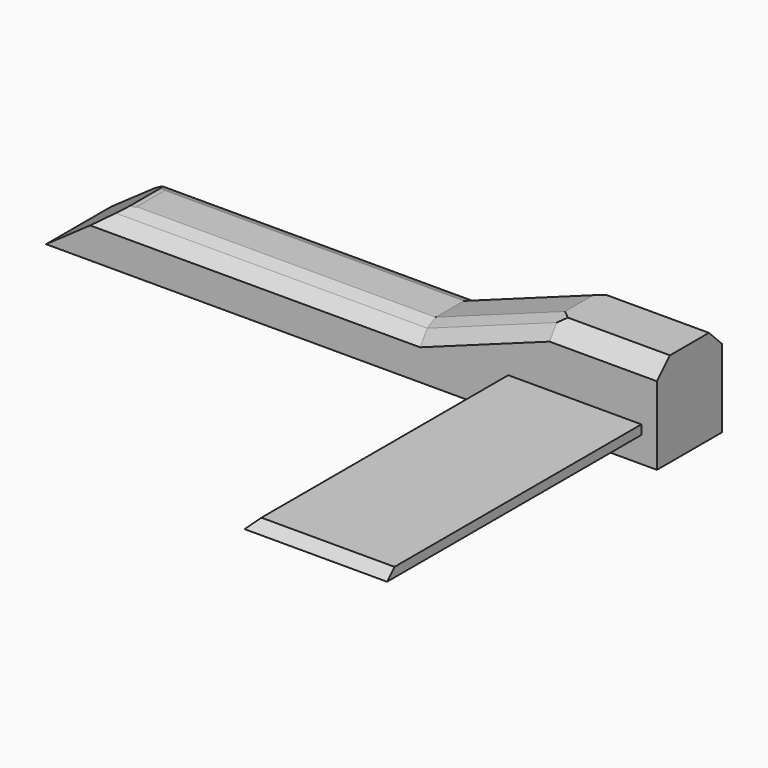
from build123d import *

# Parameters (mm, degrees)
F0_W         = 23.517049849
F0_H         = 14.5949013531
F1_DEPTH     = 25.4
F2_T4_DEPTH  = 242.6459393762
F3_SIZE      = 5.08
F4_T1_DEPTH  = 127.9476749925
F5_W         = 46.7211659998
F5_H         = 2.9200753197
F6_DEPTH     = 127
F7_T1_DEPTH  = 114.6641495789
F7_T3_DEPTH  = 72.8494651575
F7_T8_DEPTH  = 58.5750464118
F7_T14_DEPTH = 58.5750464118
F7_T20_DEPTH = 58.5750464118
F7_T26_DEPTH = 104.9770798243
F7_T32_DEPTH = 104.9770798243
F7_T38_DEPTH = 104.9770798243
F7_T44_DEPTH = 104.9770798243
F7_T50_DEPTH = 104.9770798243
F7_T56_DEPTH = 104.9770798243
F7_T62_DEPTH = 58.5750464118
F7_T68_DEPTH = 58.5750464118
F7_T74_DEPTH = 58.5750464118
F7_T81_DEPTH = 104.9770798243
F7_T86_DEPTH = 58.5750464118
F7_T94_DEPTH = 104.9770798243
F7_T99_DEPTH = 58.5750464118


# Not quite as in the source:
# - a fillet or chamfer that OpenCascade refuses, or shapes differently, is made with other operations: its cross-section is extruded or revolved along the edge and cut away or added


with BuildPart() as f1:
    # F0 (on Front) → F1 (new body)
    with BuildSketch(Plane.XZ):
        with Locations((-103.8943566382, 7.2974506766)):
            Rectangle(F0_W, F0_H)
        Polygon((-92.1358317137, 0), (0, 0), (0, 14.7395525128), (-92.1358317137, 14.7395525128), (-92.1358317137, 14.5949013531), align=None)
        Polygon((0, 0), (76.3533711433, 0), (76.3533711433, 29.4791050255), (0, 29.4791050255), (0, 14.7395525128), align=None)
    extrude(amount=F1_DEPTH)

    # F2: chamfer of 15.24 x 41.8715558725 on 1 edges, made by hand


with BuildPart() as f2_tool2:
    # F2_s3 → F2_t4 (new body)
    with BuildSketch(Plane.XZ.offset(-108.6229696881)):
        Polygon((41.8715558725, 29.4791050255), (0, 14.2391050255), (0, 29.4791050255), align=None)
    extrude(amount=F2_T4_DEPTH)

    split(bisect_by=Plane.XY.offset(14.7395525128), keep=Keep.TOP)


with BuildPart() as f1_1:
    add(f1.part)

    # F2_t1: cut F2_tool2
    add(f2_tool2.part, mode=Mode.SUBTRACT)

    # F3
    f3_edges = [f1_1.edges().sort_by_distance(p)[0] for p in [
        (-45.380432, -25.4, 14.739553),
        (-45.380432, 0, 14.739553),
        (59.112464, -25.4, 29.479105),
        (21.623262, -25.4, 22.109329),
        (21.623262, 0, 22.109329),
        (59.112464, 0, 29.479105),
    ]]
    chamfer(f3_edges, length=F3_SIZE)

    # F4: chamfer of 15.24 x 21.7649756227 on 1 edges, made by hand

    # F4_s2 → F4_t1 (cut)
    with BuildSketch(Plane.XZ.offset(-51.2738374963)):
        Polygon((-115.6528815627, -0.6450986469), (-93.88790594, 14.5949013531), (-115.6528815627, 14.5949013531), align=None)
    extrude(amount=F4_T1_DEPTH, mode=Mode.SUBTRACT)

    # F5 (on face) → F6 (join)
    with BuildSketch(Plane(origin=(0, 0, 0), x_dir=(-1, 0, 0), z_dir=(0, 1, 0))):
        with Locations((-48.1185736135, 9.490238037)):
            Rectangle(F5_W, F5_H)
    extrude(amount=-F6_DEPTH)

    # F7: chamfer of 5.08 on 6 edges, made by hand

    # F7_s2 → F7_t1 (cut)
    with BuildSketch(Plane.XZ.offset(25.4)):
        with BuildLine():
            Line((29.9816747115, 11.0939597948), (24.6143065156, 5.7265915989))
            Line((24.6143065156, 5.7265915989), (24.5127065156, 5.7265915989))
            ThreePointArc((24.5127065156, 5.7265915989), (24.6563906136, 8.3384336478), (24.6563906136, 10.9502756968))
            Line((24.6563906136, 10.9502756968), (24.7579906136, 11.0518756968))
            ThreePointArc((24.7579906136, 11.0518756968), (27.3698326625, 11.0518756968), (29.9816747115, 11.1955597948))
            Line((29.9816747115, 11.1955597948), (29.9816747115, 11.0939597948))
        make_face()
    extrude(amount=F7_T1_DEPTH, mode=Mode.SUBTRACT)

    # F7_s4 → F7_t3 (cut)
    with BuildSketch(Plane.YZ.offset(11.6938410347)):
        with BuildLine():
            Line((-121.7763159021, 11.0939597948), (-127.1436840979, 5.7265915989))
            Line((-127.1436840979, 5.7265915989), (-127.2452840979, 5.7265915989))
            ThreePointArc((-127.2452840979, 5.7265915989), (-127.1016, 8.3384336478), (-127.1016, 10.9502756968))
            Line((-127.1016, 10.9502756968), (-127, 11.0518756968))
            ThreePointArc((-127, 11.0518756968), (-124.388157951, 11.0518756968), (-121.7763159021, 11.1955597948))
            Line((-121.7763159021, 11.1955597948), (-121.7763159021, 11.0939597948))
        make_face()
    extrude(amount=F7_T3_DEPTH, mode=Mode.SUBTRACT)


with BuildPart() as f7_tool6:
    # F7_s7 → F7_t8 (new body)
    with BuildSketch(Plane(origin=(0.563938989, 0, 0.2052570059), x_dir=(0, 1, 0), z_dir=(0.9396926208, 0, 0.3420201433))):
        with BuildLine():
            Line((-7.3719372179, 13.4581431925), (-3.4043701274, 11.814723094))
            Line((-3.4043701274, 11.814723094), (-3.3325280785, 11.886565143))
            ThreePointArc((-3.3325280785, 11.886565143), (-4.1978357766, 12.6419017936), (-5.008157951, 13.452223968))
            Line((-5.008157951, 13.452223968), (-5.08, 13.4819819191))
            ThreePointArc((-5.08, 13.4819819191), (-6.2259686089, 13.4819819191), (-7.3719372179, 13.5597431925))
            Line((-7.3719372179, 13.5597431925), (-7.3719372179, 13.4581431925))
        make_face()
    extrude(amount=F7_T8_DEPTH)

    split(bisect_by=Plane.XY.offset(14.7395525128), keep=Keep.BOTTOM)

    split(bisect_by=Plane(origin=(0, 4.8297762564, 4.8297762564), x_dir=(1, 0, 0), z_dir=(0, 0.7071067812, 0.7071067812)), keep=Keep.TOP)


with BuildPart() as f1_2:
    add(f1_1.part)

    # F7_t5: cut F7_tool6
    add(f7_tool6.part, mode=Mode.SUBTRACT)


with BuildPart() as f7_tool12:
    # F7_s13 → F7_t14 (new body)
    with BuildSketch(Plane(origin=(0.563938989, 0, 0.2052570059), x_dir=(0, 1, 0), z_dir=(0.9396926208, 0, 0.3420201433))):
        with BuildLine():
            Line((-7.3719372179, 13.4581431925), (-3.4043701274, 11.814723094))
            Line((-3.4043701274, 11.814723094), (-3.3325280785, 11.886565143))
            ThreePointArc((-3.3325280785, 11.886565143), (-4.1978357766, 12.6419017936), (-5.008157951, 13.452223968))
            Line((-5.008157951, 13.452223968), (-5.08, 13.4819819191))
            ThreePointArc((-5.08, 13.4819819191), (-6.2259686089, 13.4819819191), (-7.3719372179, 13.5597431925))
            Line((-7.3719372179, 13.5597431925), (-7.3719372179, 13.4581431925))
        make_face()
    extrude(amount=F7_T14_DEPTH)

    split(bisect_by=Plane.XY.offset(14.7395525128), keep=Keep.TOP)

    split(bisect_by=Plane(origin=(0, 4.8297762564, 4.8297762564), x_dir=(1, 0, 0), z_dir=(0, -0.7071067812, -0.7071067812)), keep=Keep.TOP)


with BuildPart() as f1_3:
    add(f1_2.part)

    # F7_t11: cut F7_tool12
    add(f7_tool12.part, mode=Mode.SUBTRACT)


with BuildPart() as f7_tool18:
    # F7_s19 → F7_t20 (new body)
    with BuildSketch(Plane(origin=(0.563938989, 0, 0.2052570059), x_dir=(0, 1, 0), z_dir=(0.9396926208, 0, 0.3420201433))):
        with BuildLine():
            Line((-7.3719372179, 13.4581431925), (-3.4043701274, 11.814723094))
            Line((-3.4043701274, 11.814723094), (-3.3325280785, 11.886565143))
            ThreePointArc((-3.3325280785, 11.886565143), (-4.1978357766, 12.6419017936), (-5.008157951, 13.452223968))
            Line((-5.008157951, 13.452223968), (-5.08, 13.4819819191))
            ThreePointArc((-5.08, 13.4819819191), (-6.2259686089, 13.4819819191), (-7.3719372179, 13.5597431925))
            Line((-7.3719372179, 13.5597431925), (-7.3719372179, 13.4581431925))
        make_face()
    extrude(amount=F7_T20_DEPTH)

    split(bisect_by=Plane.XY.offset(14.7395525128), keep=Keep.TOP)

    split(bisect_by=Plane(origin=(0, 4.8297762564, 4.8297762564), x_dir=(1, 0, 0), z_dir=(0, 0.7071067812, 0.7071067812)), keep=Keep.TOP)


with BuildPart() as f1_4:
    add(f1_3.part)

    # F7_t17: cut F7_tool18
    add(f7_tool18.part, mode=Mode.SUBTRACT)


with BuildPart() as f7_tool24:
    # F7_s25 → F7_t26 (new body)
    with BuildSketch(Plane.YZ.offset(-97.8689716836)):
        with BuildLine():
            Line((-7.3719372179, 14.8173137862), (-3.4043701274, 13.1738936877))
            Line((-3.4043701274, 13.1738936877), (-3.3325280785, 13.2457357367))
            ThreePointArc((-3.3325280785, 13.2457357367), (-4.1978357766, 14.0010723873), (-5.008157951, 14.8113945617))
            Line((-5.008157951, 14.8113945617), (-5.08, 14.8411525128))
            ThreePointArc((-5.08, 14.8411525128), (-6.2259686089, 14.8411525128), (-7.3719372179, 14.9189137862))
            Line((-7.3719372179, 14.9189137862), (-7.3719372179, 14.8173137862))
        make_face()
    extrude(amount=F7_T26_DEPTH)

    split(bisect_by=Plane(origin=(-4.5763601417, 0, 12.5734461526), x_dir=(0, 1, 0), z_dir=(-0.3420201433, 0, 0.9396926208)), keep=Keep.TOP)

    split(bisect_by=Plane(origin=(-1.4194489068, 4.1501909595, 3.8999038195), x_dir=(-0.9461886483, -0.3236155771, 0), z_dir=(-0.2418447626, 0.7071067812, 0.6644630244)), keep=Keep.TOP)


with BuildPart() as f1_5:
    add(f1_4.part)

    # F7_t23: cut F7_tool24
    add(f7_tool24.part, mode=Mode.SUBTRACT)


with BuildPart() as f7_tool30:
    # F7_s31 → F7_t32 (new body)
    with BuildSketch(Plane.YZ.offset(-97.8689716836)):
        with BuildLine():
            Line((-7.3719372179, 14.8173137862), (-3.4043701274, 13.1738936877))
            Line((-3.4043701274, 13.1738936877), (-3.3325280785, 13.2457357367))
            ThreePointArc((-3.3325280785, 13.2457357367), (-4.1978357766, 14.0010723873), (-5.008157951, 14.8113945617))
            Line((-5.008157951, 14.8113945617), (-5.08, 14.8411525128))
            ThreePointArc((-5.08, 14.8411525128), (-6.2259686089, 14.8411525128), (-7.3719372179, 14.9189137862))
            Line((-7.3719372179, 14.9189137862), (-7.3719372179, 14.8173137862))
        make_face()
    extrude(amount=F7_T32_DEPTH)

    split(bisect_by=Plane(origin=(-4.5763601417, 0, 12.5734461526), x_dir=(0, 1, 0), z_dir=(0.3420201433, 0, -0.9396926208)), keep=Keep.TOP)

    split(bisect_by=Plane(origin=(-1.4194489068, 4.1501909595, 3.8999038195), x_dir=(-0.9461886483, -0.3236155771, 0), z_dir=(-0.2418447626, 0.7071067812, 0.6644630244)), keep=Keep.TOP)


with BuildPart() as f1_6:
    add(f1_5.part)

    # F7_t29: cut F7_tool30
    add(f7_tool30.part, mode=Mode.SUBTRACT)


with BuildPart() as f7_tool36:
    # F7_s37 → F7_t38 (new body)
    with BuildSketch(Plane.YZ.offset(-97.8689716836)):
        with BuildLine():
            Line((-7.3719372179, 14.8173137862), (-3.4043701274, 13.1738936877))
            Line((-3.4043701274, 13.1738936877), (-3.3325280785, 13.2457357367))
            ThreePointArc((-3.3325280785, 13.2457357367), (-4.1978357766, 14.0010723873), (-5.008157951, 14.8113945617))
            Line((-5.008157951, 14.8113945617), (-5.08, 14.8411525128))
            ThreePointArc((-5.08, 14.8411525128), (-6.2259686089, 14.8411525128), (-7.3719372179, 14.9189137862))
            Line((-7.3719372179, 14.9189137862), (-7.3719372179, 14.8173137862))
        make_face()
    extrude(amount=F7_T38_DEPTH)

    split(bisect_by=Plane(origin=(-4.5763601417, 0, 12.5734461526), x_dir=(0, 1, 0), z_dir=(-0.3420201433, 0, 0.9396926208)), keep=Keep.TOP)

    split(bisect_by=Plane(origin=(-1.4194489068, 4.1501909595, 3.8999038195), x_dir=(0.9461886483, 0.3236155771, 0), z_dir=(0.2418447626, -0.7071067812, -0.6644630244)), keep=Keep.TOP)


with BuildPart() as f1_7:
    add(f1_6.part)

    # F7_t35: cut F7_tool36
    add(f7_tool36.part, mode=Mode.SUBTRACT)


with BuildPart() as f7_tool42:
    # F7_s43 → F7_t44 (new body)
    with BuildSketch(Plane.YZ.offset(7.1081081408)):
        with BuildLine():
            Line((-21.9956298726, 13.1738936877), (-18.0280627821, 14.8173137862))
            Line((-18.0280627821, 14.8173137862), (-18.0280627821, 14.9189137862))
            ThreePointArc((-18.0280627821, 14.9189137862), (-19.1740313911, 14.8411525128), (-20.32, 14.8411525128))
            Line((-20.32, 14.8411525128), (-20.391842049, 14.8113945617))
            ThreePointArc((-20.391842049, 14.8113945617), (-21.2021642234, 14.0010723873), (-22.0674719215, 13.2457357367))
            Line((-22.0674719215, 13.2457357367), (-21.9956298726, 13.1738936877))
        make_face()
    extrude(amount=-F7_T44_DEPTH)

    split(bisect_by=Plane(origin=(-5.763104727, -16.8501909595, 15.8340001035), x_dir=(-0.9461886483, 0.3236155771, 0), z_dir=(0.2418447626, 0.7071067812, -0.6644630244)), keep=Keep.TOP)

    split(bisect_by=Plane(origin=(-4.5763601417, 0, 12.5734461526), x_dir=(0, 1, 0), z_dir=(-0.3420201433, 0, 0.9396926208)), keep=Keep.TOP)


with BuildPart() as f1_8:
    add(f1_7.part)

    # F7_t41: cut F7_tool42
    add(f7_tool42.part, mode=Mode.SUBTRACT)


with BuildPart() as f7_tool48:
    # F7_s49 → F7_t50 (new body)
    with BuildSketch(Plane.YZ.offset(7.1081081408)):
        with BuildLine():
            Line((-21.9956298726, 13.1738936877), (-18.0280627821, 14.8173137862))
            Line((-18.0280627821, 14.8173137862), (-18.0280627821, 14.9189137862))
            ThreePointArc((-18.0280627821, 14.9189137862), (-19.1740313911, 14.8411525128), (-20.32, 14.8411525128))
            Line((-20.32, 14.8411525128), (-20.391842049, 14.8113945617))
            ThreePointArc((-20.391842049, 14.8113945617), (-21.2021642234, 14.0010723873), (-22.0674719215, 13.2457357367))
            Line((-22.0674719215, 13.2457357367), (-21.9956298726, 13.1738936877))
        make_face()
    extrude(amount=-F7_T50_DEPTH)

    split(bisect_by=Plane(origin=(-5.763104727, -16.8501909595, 15.8340001035), x_dir=(0.9461886483, -0.3236155771, 0), z_dir=(-0.2418447626, -0.7071067812, 0.6644630244)), keep=Keep.TOP)

    split(bisect_by=Plane(origin=(-4.5763601417, 0, 12.5734461526), x_dir=(0, 1, 0), z_dir=(0.3420201433, 0, -0.9396926208)), keep=Keep.TOP)


with BuildPart() as f1_9:
    add(f1_8.part)

    # F7_t47: cut F7_tool48
    add(f7_tool48.part, mode=Mode.SUBTRACT)


with BuildPart() as f7_tool54:
    # F7_s55 → F7_t56 (new body)
    with BuildSketch(Plane.YZ.offset(7.1081081408)):
        with BuildLine():
            Line((-21.9956298726, 13.1738936877), (-18.0280627821, 14.8173137862))
            Line((-18.0280627821, 14.8173137862), (-18.0280627821, 14.9189137862))
            ThreePointArc((-18.0280627821, 14.9189137862), (-19.1740313911, 14.8411525128), (-20.32, 14.8411525128))
            Line((-20.32, 14.8411525128), (-20.391842049, 14.8113945617))
            ThreePointArc((-20.391842049, 14.8113945617), (-21.2021642234, 14.0010723873), (-22.0674719215, 13.2457357367))
            Line((-22.0674719215, 13.2457357367), (-21.9956298726, 13.1738936877))
        make_face()
    extrude(amount=-F7_T56_DEPTH)

    split(bisect_by=Plane(origin=(-5.763104727, -16.8501909595, 15.8340001035), x_dir=(0.9461886483, -0.3236155771, 0), z_dir=(-0.2418447626, -0.7071067812, 0.6644630244)), keep=Keep.TOP)

    split(bisect_by=Plane(origin=(-4.5763601417, 0, 12.5734461526), x_dir=(0, 1, 0), z_dir=(-0.3420201433, 0, 0.9396926208)), keep=Keep.TOP)


with BuildPart() as f1_10:
    add(f1_9.part)

    # F7_t53: cut F7_tool54
    add(f7_tool54.part, mode=Mode.SUBTRACT)


with BuildPart() as f7_tool60:
    # F7_s61 → F7_t62 (new body)
    with BuildSketch(Plane(origin=(0.563938989, 0, 0.2052570059), x_dir=(0, 1, 0), z_dir=(0.9396926208, 0, 0.3420201433))):
        with BuildLine():
            Line((-21.9956298726, 11.814723094), (-18.0280627821, 13.4581431925))
            Line((-18.0280627821, 13.4581431925), (-18.0280627821, 13.5597431925))
            ThreePointArc((-18.0280627821, 13.5597431925), (-19.1740313911, 13.4819819191), (-20.32, 13.4819819191))
            Line((-20.32, 13.4819819191), (-20.391842049, 13.452223968))
            ThreePointArc((-20.391842049, 13.452223968), (-21.2021642234, 12.6419017936), (-22.0674719215, 11.886565143))
            Line((-22.0674719215, 11.886565143), (-21.9956298726, 11.814723094))
        make_face()
    extrude(amount=F7_T62_DEPTH)

    split(bisect_by=Plane(origin=(0, -17.5297762564, 17.5297762564), x_dir=(1, 0, 0), z_dir=(0, 0.7071067812, -0.7071067812)), keep=Keep.TOP)

    split(bisect_by=Plane.XY.offset(14.7395525128), keep=Keep.TOP)


with BuildPart() as f1_11:
    add(f1_10.part)

    # F7_t59: cut F7_tool60
    add(f7_tool60.part, mode=Mode.SUBTRACT)


with BuildPart() as f7_tool66:
    # F7_s67 → F7_t68 (new body)
    with BuildSketch(Plane(origin=(0.563938989, 0, 0.2052570059), x_dir=(0, 1, 0), z_dir=(0.9396926208, 0, 0.3420201433))):
        with BuildLine():
            Line((-21.9956298726, 11.814723094), (-18.0280627821, 13.4581431925))
            Line((-18.0280627821, 13.4581431925), (-18.0280627821, 13.5597431925))
            ThreePointArc((-18.0280627821, 13.5597431925), (-19.1740313911, 13.4819819191), (-20.32, 13.4819819191))
            Line((-20.32, 13.4819819191), (-20.391842049, 13.452223968))
            ThreePointArc((-20.391842049, 13.452223968), (-21.2021642234, 12.6419017936), (-22.0674719215, 11.886565143))
            Line((-22.0674719215, 11.886565143), (-21.9956298726, 11.814723094))
        make_face()
    extrude(amount=F7_T68_DEPTH)

    split(bisect_by=Plane(origin=(0, -17.5297762564, 17.5297762564), x_dir=(1, 0, 0), z_dir=(0, -0.7071067812, 0.7071067812)), keep=Keep.TOP)

    split(bisect_by=Plane.XY.offset(14.7395525128), keep=Keep.BOTTOM)


with BuildPart() as f1_12:
    add(f1_11.part)

    # F7_t65: cut F7_tool66
    add(f7_tool66.part, mode=Mode.SUBTRACT)


with BuildPart() as f7_tool72:
    # F7_s73 → F7_t74 (new body)
    with BuildSketch(Plane(origin=(0.563938989, 0, 0.2052570059), x_dir=(0, 1, 0), z_dir=(0.9396926208, 0, 0.3420201433))):
        with BuildLine():
            Line((-21.9956298726, 11.814723094), (-18.0280627821, 13.4581431925))
            Line((-18.0280627821, 13.4581431925), (-18.0280627821, 13.5597431925))
            ThreePointArc((-18.0280627821, 13.5597431925), (-19.1740313911, 13.4819819191), (-20.32, 13.4819819191))
            Line((-20.32, 13.4819819191), (-20.391842049, 13.452223968))
            ThreePointArc((-20.391842049, 13.452223968), (-21.2021642234, 12.6419017936), (-22.0674719215, 11.886565143))
            Line((-22.0674719215, 11.886565143), (-21.9956298726, 11.814723094))
        make_face()
    extrude(amount=F7_T74_DEPTH)

    split(bisect_by=Plane(origin=(0, -17.5297762564, 17.5297762564), x_dir=(1, 0, 0), z_dir=(0, -0.7071067812, 0.7071067812)), keep=Keep.TOP)

    split(bisect_by=Plane.XY.offset(14.7395525128), keep=Keep.TOP)


with BuildPart() as f1_13:
    add(f1_12.part)

    # F7_t71: cut F7_tool72
    add(f7_tool72.part, mode=Mode.SUBTRACT)


with BuildPart() as f7_tool79:
    # F7_s80 → F7_t81 (new body)
    with BuildSketch(Plane.YZ.offset(-97.8689716836)):
        with BuildLine():
            Line((-7.3719372179, 14.8173137862), (-3.4043701274, 13.1738936877))
            Line((-3.4043701274, 13.1738936877), (-3.3325280785, 13.2457357367))
            ThreePointArc((-3.3325280785, 13.2457357367), (-4.1978357766, 14.0010723873), (-5.008157951, 14.8113945617))
            Line((-5.008157951, 14.8113945617), (-5.08, 14.8411525128))
            ThreePointArc((-5.08, 14.8411525128), (-6.2259686089, 14.8411525128), (-7.3719372179, 14.9189137862))
            Line((-7.3719372179, 14.9189137862), (-7.3719372179, 14.8173137862))
        make_face()
    extrude(amount=F7_T81_DEPTH)

    split(bisect_by=Plane(origin=(-4.5763601417, 0, 12.5734461526), x_dir=(0, 1, 0), z_dir=(0.3420201433, 0, -0.9396926208)), keep=Keep.TOP)

    split(bisect_by=Plane(origin=(-1.4194489068, 4.1501909595, 3.8999038195), x_dir=(0.9461886483, 0.3236155771, 0), z_dir=(0.2418447626, -0.7071067812, -0.6644630244)), keep=Keep.TOP)


with BuildPart() as f7_tool84:
    # F7_s85 → F7_t86 (new body)
    with BuildSketch(Plane(origin=(0.563938989, 0, 0.2052570059), x_dir=(0, 1, 0), z_dir=(0.9396926208, 0, 0.3420201433))):
        with BuildLine():
            Line((-7.3719372179, 13.4581431925), (-3.4043701274, 11.814723094))
            Line((-3.4043701274, 11.814723094), (-3.3325280785, 11.886565143))
            ThreePointArc((-3.3325280785, 11.886565143), (-4.1978357766, 12.6419017936), (-5.008157951, 13.452223968))
            Line((-5.008157951, 13.452223968), (-5.08, 13.4819819191))
            ThreePointArc((-5.08, 13.4819819191), (-6.2259686089, 13.4819819191), (-7.3719372179, 13.5597431925))
            Line((-7.3719372179, 13.5597431925), (-7.3719372179, 13.4581431925))
        make_face()
    extrude(amount=F7_T86_DEPTH)

    split(bisect_by=Plane.XY.offset(14.7395525128), keep=Keep.BOTTOM)

    split(bisect_by=Plane(origin=(0, 4.8297762564, 4.8297762564), x_dir=(1, 0, 0), z_dir=(0, -0.7071067812, -0.7071067812)), keep=Keep.TOP)


with BuildPart() as f7_tool79_1:
    add(f7_tool79.part)

    # F7_t89: intersect F7_tool84
    add(f7_tool84.part, mode=Mode.INTERSECT)


with BuildPart() as f1_14:
    add(f1_13.part)

    # F7_t77: cut F7_tool79
    add(f7_tool79_1.part, mode=Mode.SUBTRACT)


with BuildPart() as f7_tool92:
    # F7_s93 → F7_t94 (new body)
    with BuildSketch(Plane.YZ.offset(7.1081081408)):
        with BuildLine():
            Line((-21.9956298726, 13.1738936877), (-18.0280627821, 14.8173137862))
            Line((-18.0280627821, 14.8173137862), (-18.0280627821, 14.9189137862))
            ThreePointArc((-18.0280627821, 14.9189137862), (-19.1740313911, 14.8411525128), (-20.32, 14.8411525128))
            Line((-20.32, 14.8411525128), (-20.391842049, 14.8113945617))
            ThreePointArc((-20.391842049, 14.8113945617), (-21.2021642234, 14.0010723873), (-22.0674719215, 13.2457357367))
            Line((-22.0674719215, 13.2457357367), (-21.9956298726, 13.1738936877))
        make_face()
    extrude(amount=-F7_T94_DEPTH)

    split(bisect_by=Plane(origin=(-5.763104727, -16.8501909595, 15.8340001035), x_dir=(-0.9461886483, 0.3236155771, 0), z_dir=(0.2418447626, 0.7071067812, -0.6644630244)), keep=Keep.TOP)

    split(bisect_by=Plane(origin=(-4.5763601417, 0, 12.5734461526), x_dir=(0, 1, 0), z_dir=(0.3420201433, 0, -0.9396926208)), keep=Keep.TOP)


with BuildPart() as f7_tool97:
    # F7_s98 → F7_t99 (new body)
    with BuildSketch(Plane(origin=(0.563938989, 0, 0.2052570059), x_dir=(0, 1, 0), z_dir=(0.9396926208, 0, 0.3420201433))):
        with BuildLine():
            Line((-21.9956298726, 11.814723094), (-18.0280627821, 13.4581431925))
            Line((-18.0280627821, 13.4581431925), (-18.0280627821, 13.5597431925))
            ThreePointArc((-18.0280627821, 13.5597431925), (-19.1740313911, 13.4819819191), (-20.32, 13.4819819191))
            Line((-20.32, 13.4819819191), (-20.391842049, 13.452223968))
            ThreePointArc((-20.391842049, 13.452223968), (-21.2021642234, 12.6419017936), (-22.0674719215, 11.886565143))
            Line((-22.0674719215, 11.886565143), (-21.9956298726, 11.814723094))
        make_face()
    extrude(amount=F7_T99_DEPTH)

    split(bisect_by=Plane(origin=(0, -17.5297762564, 17.5297762564), x_dir=(1, 0, 0), z_dir=(0, 0.7071067812, -0.7071067812)), keep=Keep.TOP)

    split(bisect_by=Plane.XY.offset(14.7395525128), keep=Keep.BOTTOM)


with BuildPart() as f7_tool92_1:
    add(f7_tool92.part)

    # F7_t102: intersect F7_tool97
    add(f7_tool97.part, mode=Mode.INTERSECT)


with BuildPart() as f1_15:
    add(f1_14.part)

    # F7_t90: cut F7_tool92
    add(f7_tool92_1.part, mode=Mode.SUBTRACT)


solid = f1_15.part
